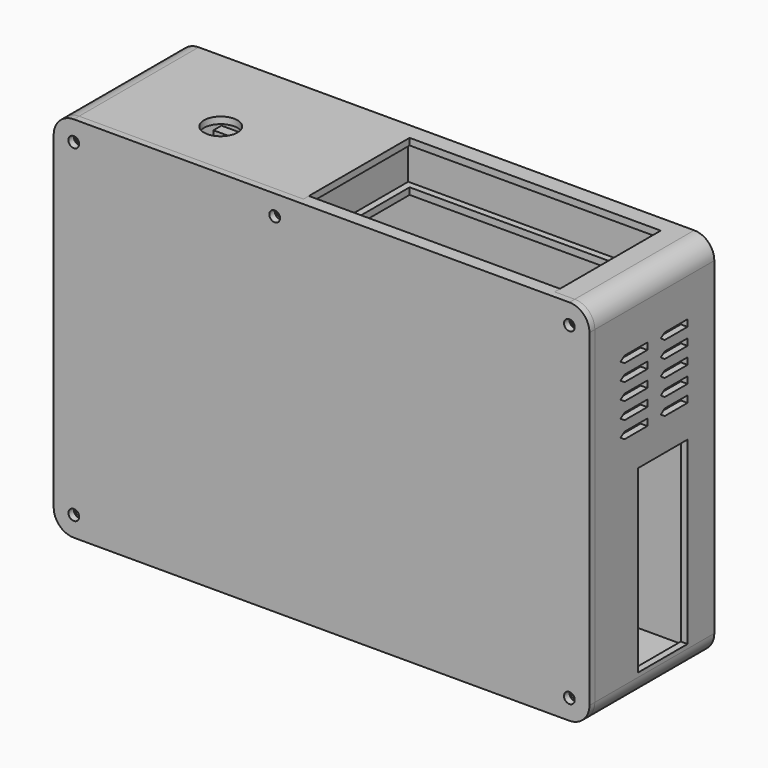
from build123d import *

# Parameters (mm, degrees)
F1_DEPTH  = 3
F3_DEPTH  = 41.6
F5_W      = 75
F5_H      = 39.6
F6_DEPTH  = 19.9
F4_R      = 3
F7_DEPTH  = 10
F8_R      = 1.25
F9_DEPTH  = 10
F12_DEPTH = 3
F14_DEPTH = 2
F16_R     = 2.5
F17_DEPTH = 2
F18_R     = 3
F18_R_2   = 3.68402633
F19_DEPTH = 4
F20_R     = 1.1
F21_DEPTH = 7
F22_W     = 17.65
F22_H     = 27.99
F23_DEPTH = 3
F25_DEPTH = 2
F27_DEPTH = 3
F28_D     = 2.2
F28_DEPTH = 6.001
F29_R     = 4
F30_DEPTH = 8
F31_R     = 1.6
F32_DEPTH = 3
F33_R     = 1.1
F34_DEPTH = 11
F35_R     = 5
F36_DEPTH = 2
F38_DEPTH = 8
F40_DEPTH = 2
F42_DEPTH = 2
F43_R     = 1.11
F44_DEPTH = 10
F45_R     = 1.6
F46_DEPTH = 2
F47_W     = 75
F47_H     = 2
F47_W_2   = 2
F47_H_2   = 85
F47_W_3   = 140
F47_W_4   = 41
F48_DEPTH = 2


with BuildPart() as f1:
    # F0 (on Front) → F1 (new body)
    with BuildSketch(Plane.XZ):
        with BuildLine():
            ThreePointArc((0, 6), (1.7573593129, 1.7573593129), (6, 0))
            Line((6, 0), (154, 0))
            ThreePointArc((154, 0), (158.2426406871, 1.7573593129), (160, 6))
            Line((160, 6), (160, 104))
            ThreePointArc((160, 104), (158.2426406871, 108.2426406871), (154, 110))
            Line((154, 110), (6, 110))
            ThreePointArc((6, 110), (1.7573593129, 108.2426406871), (0, 104))
            Line((0, 104), (0, 6))
        make_face()
    extrude(amount=F1_DEPTH)

    # F2 (on face) → F3 (join)
    with BuildSketch(Plane.XZ.offset(3)):
        with BuildLine():
            Line((154, 110), (6, 110))
            ThreePointArc((6, 110), (1.7573593129, 108.2426406871), (0, 104))
            Line((0, 104), (0, 95))
            Line((0, 95), (0, 6))
            ThreePointArc((0, 6), (1.7573593129, 1.7573593129), (6, 0))
            Line((6, 0), (84.0278342366, 0))
            Line((84.0278342366, 0), (154, 0))
            ThreePointArc((154, 0), (158.2426406871, 1.7573593129), (160, 6))
            Line((160, 6), (160, 95))
            Line((160, 95), (160, 104))
            ThreePointArc((160, 104), (158.2426406871, 108.2426406871), (154, 110))
        make_face()
        with BuildLine():
            Line((2, 10), (2, 95))
            Line((2, 95), (10, 95))
            Line((10, 95), (10, 103))
            ThreePointArc((10, 103), (11.4644660941, 106.5355339059), (15, 108))
            Line((15, 108), (56, 108))
            ThreePointArc((56, 108), (59.5355339059, 106.5355339059), (61, 103))
            Line((61, 103), (61, 100))
            ThreePointArc((61, 100), (62.4644660941, 96.4644660941), (66, 95))
            Line((66, 95), (158, 95))
            Line((158, 95), (158, 6))
            ThreePointArc((158, 6), (156.8284271247, 3.1715728753), (154, 2))
            Line((154, 2), (10, 2))
            Line((10, 2), (10, 6))
            ThreePointArc((10, 6), (8.8284271247, 8.8284271247), (6, 10))
            Line((6, 10), (2, 10))
        make_face(mode=Mode.SUBTRACT)
        Polygon((80, 108), (150, 108), (150, 97), (71, 97), (71, 108), align=None, mode=Mode.SUBTRACT)
    extrude(amount=F3_DEPTH)

    # F5 (on face) → F6 (cut)
    with BuildSketch(Plane.XY.offset(110)):
        with Locations((110.5, -24.8)):
            Rectangle(F5_W, F5_H)
    extrude(amount=-F6_DEPTH, mode=Mode.SUBTRACT)

    # F4 (on Front) → F7 (join)
    with BuildSketch(Plane.XZ):
        with Locations((72.5, 58.5)):
            Circle(F4_R)
        with Locations((130.5, 58.5)):
            Circle(F4_R)
        with Locations((130.5, 9.5)):
            Circle(F4_R)
        with Locations((72.5, 9.5)):
            Circle(F4_R)
    extrude(amount=F7_DEPTH)

    # F8 (on face) → F9 (cut, through all)
    with BuildSketch(Plane.XZ.offset(10)):
        with Locations((72.5, 58.5)):
            Circle(F8_R)
        with Locations((130.5, 58.5)):
            Circle(F8_R)
        with Locations((130.5, 9.5)):
            Circle(F8_R)
        with Locations((72.5, 9.5)):
            Circle(F8_R)
    extrude(amount=-F9_DEPTH, mode=Mode.SUBTRACT)

    # F13 (on face) → F14 (cut, through all)
    with BuildSketch(Plane.YZ.offset(160)):
        Polygon((-28.5, 44.5), (-28.5, 7.25), (-10, 7.25), (-10, 16.25), (-10, 45), (-10, 53), (-10, 61), (-28.5, 61), align=None)
    extrude(amount=-F14_DEPTH, mode=Mode.SUBTRACT)

    # F15 (on face) + F16 (on face) → F17 (cut, through all)
    with BuildSketch(Plane(origin=(0, 0, 0), x_dir=(1, 0, 0), z_dir=(0, 0, -1))):
        Polygon((36, 27), (23, 27), (23, 17), (29.5, 17), (36, 17), align=None)
        Polygon((86.1, 19), (73.1, 19), (73.1, 9), (79.6, 9), (86.1, 9), align=None)
        Polygon((91, 21), (91, 9), (102, 9), (113, 9), (113, 21), align=None)
    with BuildSketch(Plane(origin=(0, 0, 0), x_dir=(1, 0, 0), z_dir=(0, 0, -1))):
        with Locations((27.5, 35)):
            Circle(F16_R)
        with Locations((52.5, 23)):
            Circle(F16_R)
    extrude(amount=-F17_DEPTH, mode=Mode.SUBTRACT)

    # F29 (on face) → F30 (join)
    with BuildSketch(Plane.XZ.offset(3)):
        with BuildLine():
            Line((10, 98), (15, 98))
            ThreePointArc((15, 98), (18.5355339059, 99.4644660941), (20, 103))
            Line((20, 103), (20, 108))
            Line((20, 108), (15, 108))
            ThreePointArc((15, 108), (11.4644660941, 106.5355339059), (10, 103))
            Line((10, 103), (10, 98))
        make_face()
        with BuildLine():
            Line((51, 108), (51, 103))
            ThreePointArc((51, 103), (52.4644660941, 99.4644660941), (56, 98))
            Line((56, 98), (61.417424305, 98))
            ThreePointArc((61.417424305, 98), (61.1054684353, 98.9784517816), (61, 100))
            Line((61, 100), (61, 103))
            ThreePointArc((61, 103), (59.5355339059, 106.5355339059), (56, 108))
            Line((56, 108), (51, 108))
        make_face()
        with BuildLine():
            ThreePointArc((52, 6), (48, 10), (44, 6))
            Line((44, 6), (44, 2))
            Line((44, 2), (52, 2))
            Line((52, 2), (52, 6))
        make_face()
        with Locations((8, 38)):
            Circle(F29_R)
        with Locations((48, 38)):
            Circle(F29_R)
        with BuildLine():
            Line((18, 2), (18, 6))
            ThreePointArc((18, 6), (16.8284271247, 8.8284271247), (14, 10))
            Line((14, 10), (6, 10))
            ThreePointArc((6, 10), (8.8284271247, 8.8284271247), (10, 6))
            Line((10, 6), (10, 2))
            Line((10, 2), (18, 2))
        make_face()
    extrude(amount=F30_DEPTH)

    # F33 (on offset) → F34 (cut, through all)
    with BuildSketch(Plane.XZ.offset(11)):
        with Locations((15.45, 102.55)):
            Circle(F33_R)
        with Locations((55.5, 102.5)):
            Circle(F33_R)
        with Locations((48, 38)):
            Circle(F33_R)
        with Locations((48, 6)):
            Circle(F33_R)
        with Locations((14, 6)):
            Circle(F33_R)
        with Locations((8, 38)):
            Circle(F33_R)
    extrude(amount=-F34_DEPTH, mode=Mode.SUBTRACT)

    # F35 (on face) → F36 (cut, through all)
    with BuildSketch(Plane.XY.offset(110)):
        with Locations((35, -28)):
            Circle(F35_R)
    extrude(amount=-F36_DEPTH, mode=Mode.SUBTRACT)

    # F37 (on face) → F38 (join)
    with BuildSketch(Plane.XZ.offset(44.6)):
        with BuildLine():
            Line((150, 2), (154, 2))
            ThreePointArc((154, 2), (156.8284271247, 3.1715728753), (158, 6))
            Line((158, 6), (158, 10))
            Line((158, 10), (154, 10))
            ThreePointArc((154, 10), (151.1715728753, 8.8284271247), (150, 6))
            Line((150, 6), (150, 2))
        make_face()
    extrude(amount=-F38_DEPTH)

    # F39 (on face) → F40 (cut, through all)
    with BuildSketch(Plane(origin=(0, 0, 0), x_dir=(0, -1, 0), z_dir=(-1, 0, 0))):
        Polygon((10, 21), (10, 19), (18.5, 19), (20, 20), (18.5, 21), align=None)
        Polygon((18.5, 24), (20, 25), (18.5, 26), (10, 26), (10, 24), align=None)
        Polygon((18.5, 29), (20, 30), (18.5, 31), (10, 31), (10, 29), align=None)
        Polygon((18.5, 34), (20, 35), (18.5, 36), (10, 36), (10, 34), align=None)
        Polygon((18.5, 39), (20, 40), (18.5, 41), (10, 41), (10, 39), align=None)
        Polygon((18.5, 44), (20, 45), (18.5, 46), (10, 46), (10, 44), align=None)
        Polygon((18.5, 49), (20, 50), (18.5, 51), (10, 51), (10, 49), align=None)
        Polygon((18.5, 54), (20, 55), (18.5, 56), (10, 56), (10, 54), align=None)
        Polygon((18.5, 59), (20, 60), (18.5, 61), (10, 61), (10, 59), align=None)
        Polygon((18.5, 64), (20, 65), (18.5, 66), (10, 66), (10, 64), align=None)
        Polygon((18.5, 69), (20, 70), (18.5, 71), (10, 71), (10, 69), align=None)
        Polygon((18.5, 74), (20, 75), (18.5, 76), (10, 76), (10, 74), align=None)
        Polygon((18.5, 79), (20, 80), (18.5, 81), (10, 81), (10, 79), align=None)
        Polygon((18.5, 84), (20, 85), (18.5, 86), (10, 86), (10, 84), align=None)
        Polygon((18.5, 89), (20, 90), (18.5, 91), (10, 91), (10, 89), align=None)
        Polygon((33.5, 19), (35, 20), (33.5, 21), (25, 21), (25, 19), align=None)
        Polygon((33.5, 24), (35, 25), (33.5, 26), (25, 26), (25, 24), align=None)
        Polygon((33.5, 29), (35, 30), (33.5, 31), (25, 31), (25, 29), align=None)
        Polygon((33.5, 34), (35, 35), (33.5, 36), (25, 36), (25, 34), align=None)
        Polygon((33.5, 39), (35, 40), (33.5, 41), (25, 41), (25, 39), align=None)
        Polygon((33.5, 44), (35, 45), (33.5, 46), (25, 46), (25, 44), align=None)
        Polygon((33.5, 49), (35, 50), (33.5, 51), (25, 51), (25, 49), align=None)
        Polygon((33.5, 54), (35, 55), (33.5, 56), (25, 56), (25, 54), align=None)
        Polygon((33.5, 59), (35, 60), (33.5, 61), (25, 61), (25, 59), align=None)
        Polygon((33.5, 64), (35, 65), (33.5, 66), (25, 66), (25, 64), align=None)
        Polygon((33.5, 69), (35, 70), (33.5, 71), (25, 71), (25, 69), align=None)
        Polygon((33.5, 74), (35, 75), (33.5, 76), (25, 76), (25, 74), align=None)
        Polygon((33.5, 79), (35, 80), (33.5, 81), (25, 81), (25, 79), align=None)
        Polygon((33.5, 84), (35, 85), (33.5, 86), (25, 86), (25, 84), align=None)
        Polygon((33.5, 89), (35, 90), (33.5, 91), (25, 91), (25, 89), align=None)
    extrude(amount=-F40_DEPTH, mode=Mode.SUBTRACT)

    # F41 (on face) → F42 (cut, through all)
    with BuildSketch(Plane.YZ.offset(160)):
        Polygon((-10, 72.6383287907), (-18.5, 72.6383287907), (-20, 71.6383287907), (-18.5, 70.6383287907), (-10, 70.6383287907), align=None)
        Polygon((-20, 76.6383287907), (-18.5, 75.6383287907), (-10, 75.6383287907), (-10, 77.6383287907), (-18.5, 77.6383287907), align=None)
        Polygon((-20, 81.6383287907), (-18.5, 80.6383287907), (-10, 80.6383287907), (-10, 82.6383287907), (-18.5, 82.6383287907), align=None)
        Polygon((-20, 86.6383287907), (-18.5, 85.6383287907), (-10, 85.6383287907), (-10, 87.6383287907), (-18.5, 87.6383287907), align=None)
        Polygon((-20, 91.6383287907), (-18.5, 90.6383287907), (-10, 90.6383287907), (-10, 92.6383287907), (-18.5, 92.6383287907), align=None)
        Polygon((-35, 71.6383287907), (-33.5, 70.6383287907), (-25, 70.6383287907), (-25, 72.6383287907), (-33.5, 72.6383287907), align=None)
        Polygon((-35, 76.6383287907), (-33.5, 75.6383287907), (-25, 75.6383287907), (-25, 77.6383287907), (-33.5, 77.6383287907), align=None)
        Polygon((-35, 81.6383287907), (-33.5, 80.6383287907), (-25, 80.6383287907), (-25, 82.6383287907), (-33.5, 82.6383287907), align=None)
        Polygon((-35, 86.6383287907), (-33.5, 85.6383287907), (-25, 85.6383287907), (-25, 87.6383287907), (-33.5, 87.6383287907), align=None)
        Polygon((-35, 91.6383287907), (-33.5, 90.6383287907), (-25, 90.6383287907), (-25, 92.6383287907), (-33.5, 92.6383287907), align=None)
    extrude(amount=-F42_DEPTH, mode=Mode.SUBTRACT)

    # F43 (on face) → F44 (cut)
    with BuildSketch(Plane.XZ.offset(44.6)):
        with Locations((6, 104)):
            Circle(F43_R)
        with Locations((66, 104)):
            Circle(F43_R)
        with Locations((154, 104)):
            Circle(F43_R)
        with Locations((154, 6)):
            Circle(F43_R)
        with Locations((6, 6)):
            Circle(F43_R)
    extrude(amount=-F44_DEPTH, mode=Mode.SUBTRACT)


with BuildPart() as f12:
    # F11 (on offset) → F12 (new body)
    with BuildSketch(Plane.XZ.offset(11)):
        with BuildLine():
            Line((60.5, 62), (60.5, 102.5))
            ThreePointArc((60.5, 102.5), (59.0355339059, 106.0355339059), (55.5, 107.5))
            Line((55.5, 107.5), (15.45, 107.5))
            ThreePointArc((15.45, 107.5), (11.9498214331, 106.0501785669), (10.5, 102.55))
            Line((10.5, 102.55), (10.5, 94.5))
            Line((10.5, 94.5), (2.5, 94.5))
            Line((2.5, 94.5), (2.5, 10.5))
            Line((2.5, 10.5), (6, 10.5))
            ThreePointArc((6, 10.5), (9.1819805153, 9.1819805153), (10.5, 6))
            Line((10.5, 6), (10.5, 2.5))
            Line((10.5, 2.5), (55, 2.5))
            Line((55, 2.5), (55, 32.3211364448))
            Line((55, 32.3211364448), (55, 57))
            ThreePointArc((55, 57), (56.4644660941, 60.5355339059), (60, 62))
            Line((60, 62), (60.5, 62))
        make_face()
    extrude(amount=F12_DEPTH)

    # F18 (on face) → F19 (join)
    with BuildSketch(Plane.XZ.offset(14)):
        with Locations((20.675, 8.605)):
            Circle(F18_R)
        with Locations((38.325, 8.605)):
            Circle(F18_R)
        with Locations((40.93, 42.2)):
            Circle(F18_R_2)
        with Locations((18.07, 42.2)):
            Circle(F18_R_2)
    extrude(amount=F19_DEPTH)

    # F20 (on face) → F21 (cut, through all)
    with BuildSketch(Plane.XZ.offset(18)):
        with Locations((20.675, 8.605)):
            Circle(F20_R)
        with Locations((38.325, 8.605)):
            Circle(F20_R)
    extrude(amount=-F21_DEPTH, mode=Mode.SUBTRACT)

    # F22 (on face) → F23 (cut, through all)
    with BuildSketch(Plane.XZ.offset(14)):
        with Locations((29.5, 25.6)):
            Rectangle(F22_W, F22_H)
    extrude(amount=-F23_DEPTH, mode=Mode.SUBTRACT)

    # F24 (on face) → F25 (join)
    with BuildSketch(Plane.XZ.offset(18)):
        with BuildLine():
            ThreePointArc((17.1165038231, 38.6415038231), (18.07, 42.2), (21.6284961769, 43.1534961769))
            ThreePointArc((21.6284961769, 43.1534961769), (15.465, 44.805), (17.1165038231, 38.6415038231))
        make_face()
        with BuildLine():
            ThreePointArc((37.3715038231, 43.1534961769), (40.93, 42.2), (41.8834961769, 38.6415038231))
            ThreePointArc((41.8834961769, 38.6415038231), (43.8527345946, 39.9573068669), (44.61402633, 42.2))
            ThreePointArc((44.61402633, 42.2), (41.4108619289, 45.852508974), (37.3715038231, 43.1534961769))
        make_face()
    extrude(amount=F25_DEPTH)

    # F26 (on face) → F27 (join)
    with BuildSketch(Plane.XZ.offset(14)):
        Polygon((32.0194885135, 100.9414463043), (24.0194885135, 100.9414463043), (24.0194885135, 50.9414463043), (40.0194885135, 50.9414463043), (40.0194885135, 75.9414463043), (40.0194885135, 100.9414463043), align=None)
    extrude(amount=F27_DEPTH)

    # F28 (through all, one way)
    with BuildSketch(Plane(origin=(0, -14, 0), x_dir=(1, 0, 0), z_dir=(0, 1, 0))):
        with Locations((32.0194885135, -93.7214463043), (32.0194885135, -84.8314463043), (32.0194885135, -75.9414463043), (32.0194885135, -67.0514463043), (32.0194885135, -58.1614463043)):
            Circle(F28_D / 2)
    extrude(amount=-F28_DEPTH, mode=Mode.SUBTRACT)

    # F31 (on face) → F32 (cut)
    with BuildSketch(Plane.XZ.offset(14)):
        with Locations((15.45, 102.55)):
            Circle(F31_R)
        with Locations((55.5, 102.5)):
            Circle(F31_R)
        with Locations((48, 38)):
            Circle(F31_R)
        with Locations((48, 6)):
            Circle(F31_R)
        with Locations((14, 6)):
            Circle(F31_R)
        with Locations((8, 38)):
            Circle(F31_R)
    extrude(amount=-F32_DEPTH, mode=Mode.SUBTRACT)


with BuildPart() as f46:
    # F45 (on face) → F46 (new body)
    with BuildSketch(Plane.XZ.offset(44.6)):
        with BuildLine():
            Line((154, 110), (6, 110))
            ThreePointArc((6, 110), (1.7573593129, 108.2426406871), (0, 104))
            Line((0, 104), (0, 6))
            ThreePointArc((0, 6), (1.7573593129, 1.7573593129), (6, 0))
            Line((6, 0), (154, 0))
            ThreePointArc((154, 0), (158.2426406871, 1.7573593129), (160, 6))
            Line((160, 6), (160, 104))
            ThreePointArc((160, 104), (158.2426406871, 108.2426406871), (154, 110))
        make_face()
        with Locations((6, 6)):
            Circle(F45_R, mode=Mode.SUBTRACT)
        with Locations((154, 6)):
            Circle(F45_R, mode=Mode.SUBTRACT)
        with Locations((6, 104)):
            Circle(F45_R, mode=Mode.SUBTRACT)
        with Locations((66, 104)):
            Circle(F45_R, mode=Mode.SUBTRACT)
        with Locations((154, 104)):
            Circle(F45_R, mode=Mode.SUBTRACT)
    extrude(amount=F46_DEPTH)

    # F47 (on face) → F48 (join)
    with BuildSketch(Plane(origin=(0, -44.6, 0), x_dir=(-1, 0, 0), z_dir=(0, 1, 0))):
        with Locations((-110.5, 109)):
            Rectangle(F47_W, F47_H)
        with Locations((-157, 52.5)):
            Rectangle(F47_W_2, F47_H_2)
        with Locations((-80, 3)):
            Rectangle(F47_W_3, F47_H)
        with Locations((-35.5, 107)):
            Rectangle(F47_W_4, F47_H)
        with Locations((-3, 52.5)):
            Rectangle(F47_W_2, F47_H_2)
    extrude(amount=F48_DEPTH)


solid = Compound([f1.part, f12.part, f46.part])
